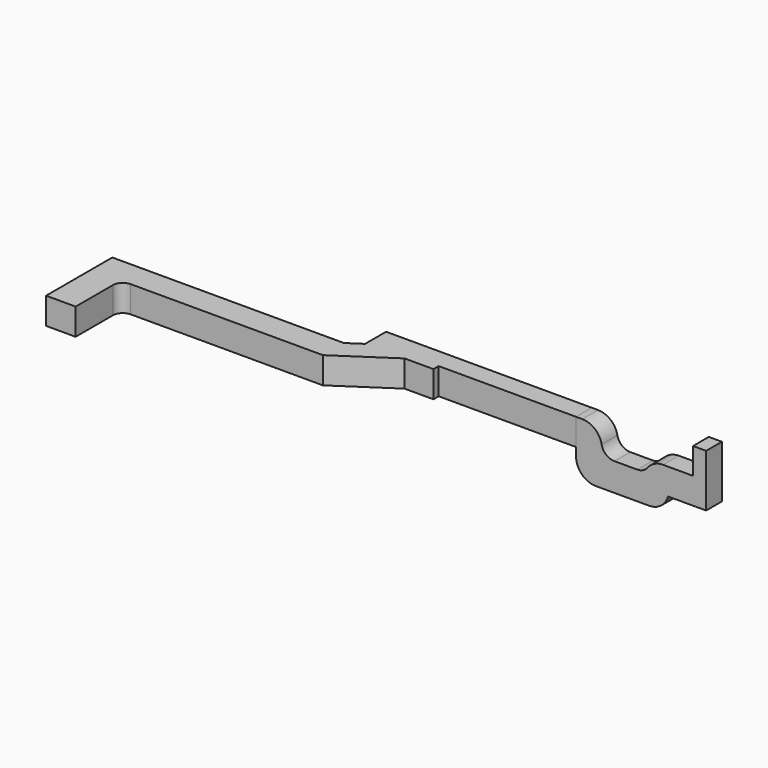
from build123d import *

# Parameters (mm, degrees)
F0_W        = 4.5
F0_H        = 8.6
F0_W_2      = 20.9
F0_H_2      = 3
F1_DEPTH    = 4.05
F0_W_3      = 19.8
F2_DEPTH    = 8.3
F3_DEPTH    = 1.88
F4_W        = 5.8
F4_H        = 2.18
F5_DEPTH    = 25
F6_T1_DEPTH = 18
F6_T3_DEPTH = 17.4287906631
F6_T5_DEPTH = 16.9987425023
F7_R        = 2
F8_R        = 1.5


# Not quite as in the source:
# - a fillet or chamfer that OpenCascade refuses, or shapes differently, is made with other operations: its cross-section is extruded or revolved along the edge and cut away or added
# - a feature names something its author has since deleted; it is built from what else it names


with BuildPart() as f1:
    # F0 (on Top) → F1 (new body)
    with BuildSketch(Plane.XY):
        with Locations((2.25, 4.3)):
            Rectangle(F0_W, F0_H)
        Polygon((0, 12.6), (0, 8.6), (4.5, 8.6), (35.25, 8.6), (35.25, 12.6), align=None)
        Polygon((35.25, 12.6), (35.25, 8.6), (43.35, 14), (37.35, 14), align=None)
        Polygon((37.35, 14), (43.35, 14), (47.76, 14), (47.76, 15), (47.76, 18), (37.35, 18), align=None)
        with Locations((58.21, 16.5)):
            Rectangle(F0_W_2, F0_H_2)
    extrude(amount=-F1_DEPTH)

    # F8
    f8_edges = [f1.edges().sort_by_distance(p)[0] for p in [
        (4.5, 8.6, -2.025),
    ]]
    fillet(f8_edges, radius=F8_R)


with BuildPart() as f2:
    # F0 (on Top) → F2 (new body)
    with BuildSketch(Plane.XY):
        with Locations((78.56, 16.5)):
            Rectangle(F0_W_3, F0_H_2)
    extrude(amount=-F2_DEPTH)

    # F0 (on Top) → F3 (join)
    with BuildSketch(Plane.XY):
        with Locations((78.56, 16.5)):
            Rectangle(F0_W_3, F0_H_2)
    extrude(amount=F3_DEPTH)

    # F4 (on face) → F5 (cut)
    with BuildSketch(Plane(origin=(0, 18, 0), x_dir=(-1, 0, 0), z_dir=(0, 1, 0))):
        with Locations((-85.56, -7.21)):
            Rectangle(F4_W, F4_H)
        Polygon((-68.66, 1.88), (-86.46, 1.88), (-86.46, -2.12), (-82.66, -2.12), (-79.1077613831, -2.12), (-79.1077613831, -4.0423134342), (-72.6052895188, -4.0423134342), (-72.6052895188, 0), (-68.66, 0), align=None)
    extrude(amount=-F5_DEPTH, mode=Mode.SUBTRACT)

    # F6: fillet of radius 3 on 4 edges, made by hand

    # F6_s2 → F6_t1 (cut)
    with BuildSketch(Plane.XZ.offset(-25.5)):
        with BuildLine():
            ThreePointArc((68.66, -5.3), (69.5386796564, -7.4213203436), (71.66, -8.3))
            Line((71.66, -8.3), (68.66, -8.3))
            Line((68.66, -8.3), (68.66, -5.3))
        make_face()
        with BuildLine():
            ThreePointArc((69.6052895188, 0), (71.7266098624, -0.8786796564), (72.6052895188, -3))
            Line((72.6052895188, -3), (72.6052895188, 0))
            Line((72.6052895188, 0), (69.6052895188, 0))
        make_face()
    extrude(amount=F6_T1_DEPTH, mode=Mode.SUBTRACT)

    # F6_s4 → F6_t3 (cut)
    with BuildSketch(Plane.XZ.offset(-25.2143953316)):
        with BuildLine():
            ThreePointArc((79.7742418674, -8.3), (81.5825559994, -7.6937418407), (82.66, -6.12))
            Line((82.66, -6.12), (82.66, -8.3))
            Line((82.66, -8.3), (79.7742418674, -8.3))
        make_face()
    extrude(amount=F6_T3_DEPTH, mode=Mode.SUBTRACT)

    # F6_s6 → F6_t5 (cut)
    with BuildSketch(Plane.XZ.offset(-24.9993712512)):
        with BuildLine():
            ThreePointArc((81.9075098835, -2.12), (80.2094315133, -2.6468380868), (79.1077613831, -4.0423134342))
            Line((79.1077613831, -4.0423134342), (79.1077613831, -2.12))
            Line((79.1077613831, -2.12), (81.9075098835, -2.12))
        make_face()
    extrude(amount=F6_T5_DEPTH, mode=Mode.SUBTRACT)

    # F7
    f7_edges = [f2.edges().sort_by_distance(p)[0] for p in [
        (72.60529, 16.5, -4.042313),
        (79.107761, 16.5, -4.042313),
    ]]
    fillet(f7_edges, radius=F7_R)


solid = Compound([f1.part, f2.part])
